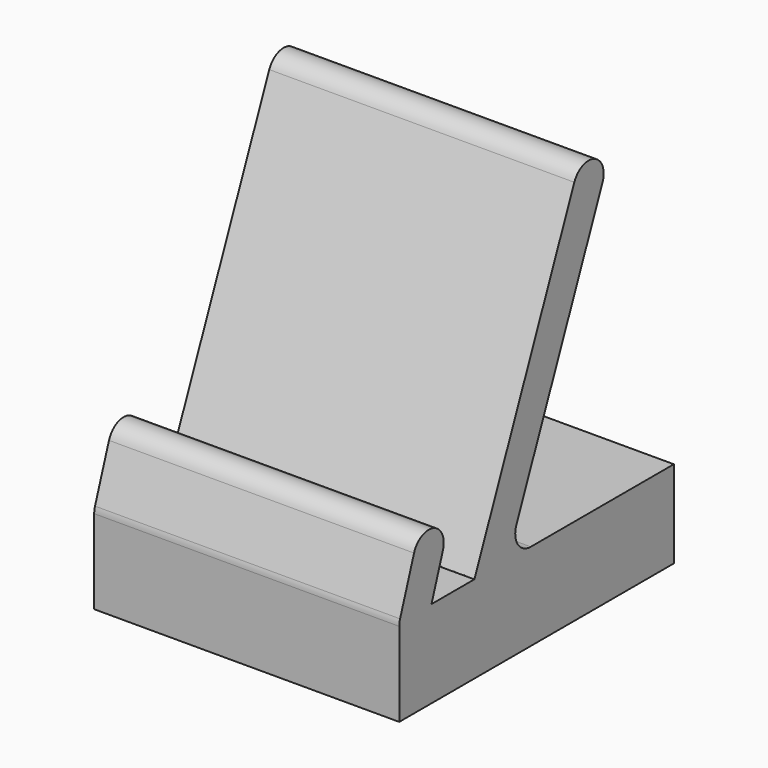
from build123d import *

# Parameters (mm, degrees)
F1_DEPTH    = 80
F2_R        = 5
F3_T1_DEPTH = 105.4
F4_T1_DEPTH = 105.4
F5_R        = 5.08


# Not quite as in the source:
# - a fillet or chamfer that OpenCascade refuses, or shapes differently, is made with other operations: its cross-section is extruded or revolved along the edge and cut away or added


with BuildPart() as f1:
    # F0 (on Right) → F1 (new body)
    with BuildSketch(Plane.YZ):
        Polygon((-65.3676100316, -25.1990987622), (-71.8711540103, -44.1121608019), (-61.2964517447, -44.1121608019), (-55.9110790118, -28.4508707515), align=None)
        Polygon((-61.2964517447, -44.1121608019), (-71.8711540103, -44.1121608019), (-71.8711540103, -67.0164749026), (18.1288459897, -67.0164749026), (18.1288459897, -44.1121608019), (-36.4091803752, -44.1121608019), (-47.0806523531, -44.1121608019), (-47.2488089486, -44.1121608019), align=None)
        Polygon((-47.220791987, -44.0451827606), (-47.2488089486, -44.1121608019), (-47.0806523531, -44.1121608019), align=None)
        Polygon((-47.2488089486, -44.031792393), (-47.2488089486, -44.1121608019), (-47.220791987, -44.0451827606), align=None)
        Polygon((-47.220791987, -44.0451827606), (-47.0806523531, -44.1121608019), (-36.4091803752, -44.1121608019), (-3.2924475957, 35.0575196106), (-12.5178559501, 38.9165143882), align=None)
    extrude(amount=F1_DEPTH)

    # F2
    f2_edges = [f1.edges().sort_by_distance(p)[0] for p in [
        (40, -71.871154, -44.112161),
    ]]
    fillet(f2_edges, radius=F2_R)

    # F3: fillet of radius 5.08 on 2 edges, made by hand

    # F3_s2 → F3_t1 (cut)
    with BuildSketch(Plane.YZ.offset(-12.7)):
        with BuildLine():
            ThreePointArc((-5.2528169427, 30.3710121665), (-5.2392727341, 34.2590522484), (-7.9789550397, 37.0178889576))
            Line((-7.9789550397, 37.0178889576), (-3.2924475957, 35.0575196106))
            Line((-3.2924475957, 35.0575196106), (-5.2528169427, 30.3710121665))
        make_face()
        with BuildLine():
            ThreePointArc((-14.4782252971, 34.2300069441), (-11.719388588, 36.9696892498), (-7.8313485061, 36.9561450412))
            Line((-7.8313485061, 36.9561450412), (-12.5178559501, 38.9165143882))
            Line((-12.5178559501, 38.9165143882), (-14.4782252971, 34.2300069441))
        make_face()
    extrude(amount=F3_T1_DEPTH, mode=Mode.SUBTRACT)

    # F4: fillet of radius 5.08 on 2 edges, made by hand

    # F4_s2 → F4_t1 (cut)
    with BuildSketch(Plane.YZ.offset(-12.7)):
        with BuildLine():
            ThreePointArc((-60.7149967698, -26.798970581), (-57.801944305, -29.3740753285), (-57.5629791823, -33.2547885096))
            Line((-57.5629791823, -33.2547885096), (-55.9110790118, -28.4508707515))
            Line((-55.9110790118, -28.4508707515), (-60.7149967698, -26.798970581))
        make_face()
        with BuildLine():
            ThreePointArc((-67.0195102022, -30.0030165203), (-64.4444054547, -27.0899640554), (-60.5636922735, -26.8509989328))
            Line((-60.5636922735, -26.8509989328), (-65.3676100316, -25.1990987622))
            Line((-65.3676100316, -25.1990987622), (-67.0195102022, -30.0030165203))
        make_face()
    extrude(amount=F4_T1_DEPTH, mode=Mode.SUBTRACT)

    # F5
    f5_edges = [f1.edges().sort_by_distance(p)[0] for p in [
        (40, -36.40918, -44.112161),
    ]]
    fillet(f5_edges, radius=F5_R)


solid = f1.part
